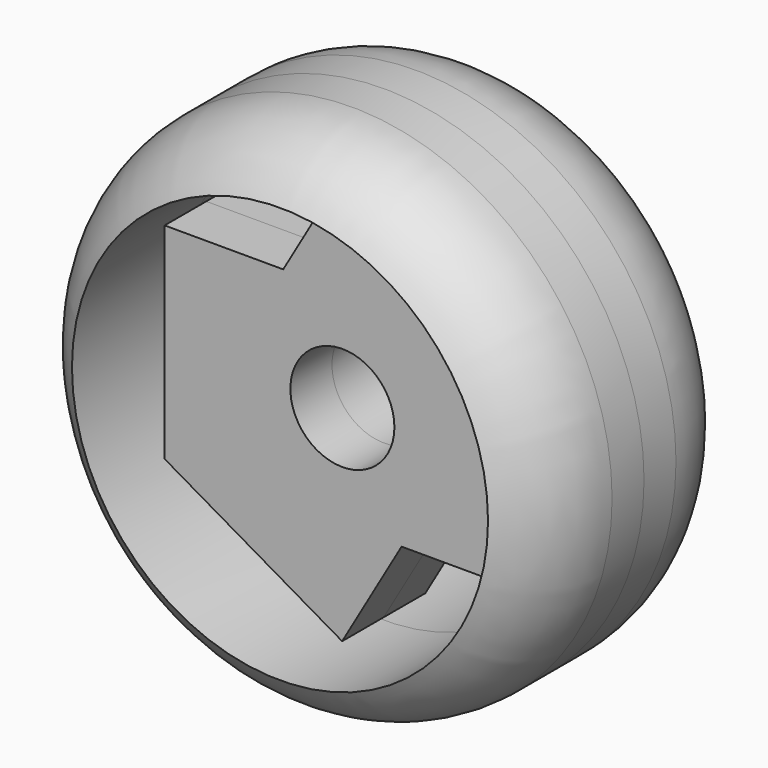
from build123d import *

# Parameters (mm, degrees)
F0_R     = 10
F1_DEPTH = 10
F0_R_2   = 50
F0_R_3   = 40
F2_DEPTH = 25


# Not quite as in the source:
# - a fillet or chamfer that OpenCascade refuses, or shapes differently, is made with other operations: its cross-section is extruded or revolved along the edge and cut away or added


with BuildPart() as f1:
    # F0 (on Front) → F1 (new body)
    with BuildSketch(Plane.XZ):
        Polygon((34.228804297, 19.707416502), (0.0472788148, 39.4967223134), (-11.3780822225, 19.7620093749), (-34.1815254822, 19.7893058113), (-34.228804297, -19.707416502), (-0.0472788148, -39.4967223134), (11.3780822225, -19.7620093749), (34.1815254822, -19.7893058113), align=None)
        Circle(F0_R, mode=Mode.SUBTRACT)
    extrude(amount=F1_DEPTH)


with BuildPart() as f2:
    # F0 (on Front) → F2 (new body)
    with BuildSketch(Plane.XZ):
        Circle(F0_R_2)
        Circle(F0_R_3, mode=Mode.SUBTRACT)
    extrude(amount=F2_DEPTH)


with BuildPart() as f3_1:
    # F3: instance of F2
    add(f2.part.mirror(Plane.XZ))

    # F4#2: fillet of radius 20 on 1 edges, made by hand

    # F4_2_s1 → F4_2_t2 (revolve, cut)
    with BuildSketch(Plane.XY):
        with BuildLine():
            ThreePointArc((50, 7.6794919243), (47.3205080757, 17.6794919243), (40, 25))
            Line((40, 25), (50, 25))
            Line((50, 25), (50, 7.6794919243))
        make_face()
    revolve(axis=Axis((0, 25, 0), (0, -1, 0)), mode=Mode.SUBTRACT)


with BuildPart() as f3_2:
    # F3: instance of F1
    add(f1.part.mirror(Plane.XZ))


with BuildPart() as f2_1:
    add(f2.part)

    # F4: fillet of radius 20 on 1 edges, made by hand

    # F4_s1 → F4_t2 (revolve, cut)
    with BuildSketch(Plane.XY):
        with BuildLine():
            ThreePointArc((50, -7.6794919243), (47.3205080757, -17.6794919243), (40, -25))
            Line((40, -25), (50, -25))
            Line((50, -25), (50, -7.6794919243))
        make_face()
    revolve(axis=Axis((0, -25, 0), (0, -1, 0)), mode=Mode.SUBTRACT)


solid = Compound([f1.part, f3_1.part, f3_2.part, f2_1.part])
